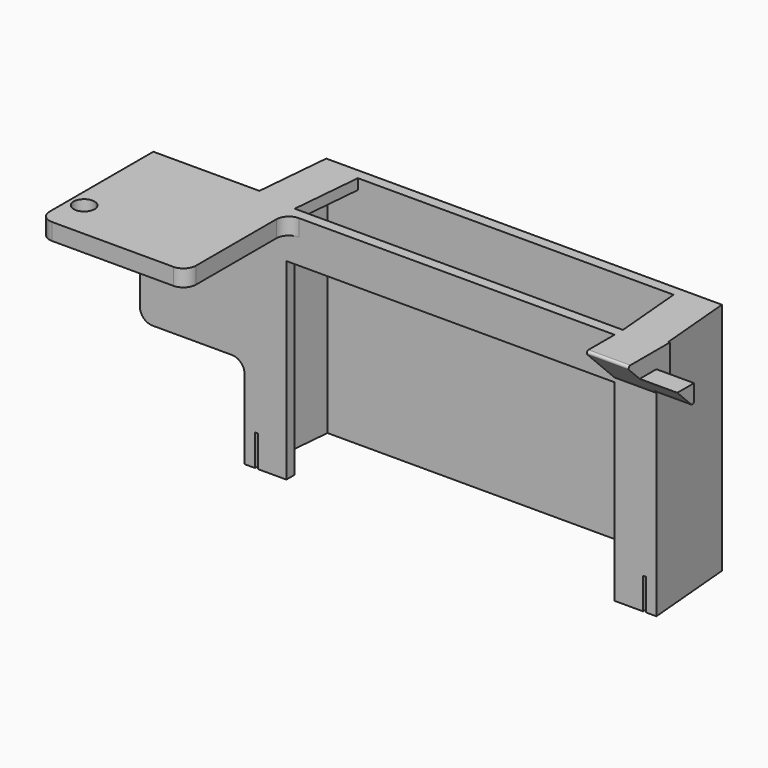
from build123d import *

# Parameters (mm, degrees)
F1_DEPTH     = 56
F3_DEPTH     = 2.5
F5_DEPTH     = 0.75
F6_SIZE      = 0.5
F7_SIZE      = 0.5
F9_DEPTH     = 7.5
F11_DEPTH    = 4
F13_DEPTH    = 30
F15_DEPTH    = 5
F16_W        = 4
F16_H        = 9
F17_DEPTH    = 9
F19_DEPTH    = 10
F20_T1_DEPTH = 25.0355339059
F20_T3_DEPTH = 10.25
F20_T5_DEPTH = 12.017766953
F21_W        = 78.4606024017
F21_H        = 2.5
F22_DEPTH    = 10
F23_R        = 2.5
F24_DEPTH    = 4
F25_R        = 3
F27_DEPTH    = 9


# Not quite as in the source:
# - a fillet or chamfer that OpenCascade refuses, or shapes differently, is made with other operations: its cross-section is extruded or revolved along the edge and cut away or added


with BuildPart() as f1:
    # F0 (on Top) → F1 (new body)
    with BuildSketch(Plane.XY):
        Polygon((-39.2303012009, -8.5), (-46.5, -8.5), (-45, 8.5), (45, 8.5), (46.5, -8.5), (39.2303012009, -8.5), (39.2303012009, -11), (49.2303012009, -11), (47.2891247303, 11), (-47.2891247303, 11), (-49.2303012009, -11), (-39.2303012009, -11), align=None)
    extrude(amount=F1_DEPTH)

    # F2 (on face) → F3 (join)
    with BuildSketch(Plane.XY.offset(56)):
        Polygon((-46.5, -8.5), (-39.2303012009, -8.5), (-37.7303012009, 8.5), (-45, 8.5), align=None)
        Polygon((46.5, -8.5), (45, 8.5), (37.7303012009, 8.5), (39.2303012009, -8.5), align=None)
    extrude(amount=-F3_DEPTH)

    # F4 (on face) → F5 (join)
    with BuildSketch(Plane(origin=(0, 0, 0), x_dir=(1, 0, 0), z_dir=(0, 0, -1))):
        Polygon((-40.7303012009, 7.75), (-40.2303012009, 8.5), (-45.5, 8.5), (-45, 7.75), align=None)
        Polygon((45, 7.75), (45.5, 8.5), (40.2303012009, 8.5), (40.7303012009, 7.75), align=None)
    extrude(amount=-F5_DEPTH)

    # F6
    f6_edges = [f1.edges().sort_by_distance(p)[0] for p in [
        (42.865151, -7.75, 0.75),
    ]]
    chamfer(f6_edges, length=F6_SIZE)

    # F7
    f7_edges = [f1.edges().sort_by_distance(p)[0] for p in [
        (-42.865151, -7.75, 0.75),
    ]]
    chamfer(f7_edges, length=F7_SIZE)

    # F8 (on face) → F9 (cut)
    with BuildSketch(Plane(origin=(0, 0, 0), x_dir=(1, 0, 0), z_dir=(0, 0, -1))):
        Polygon((-46.7205882353, 11), (-46.5, 8.5), (-45.8406183737, 8.5), (-46.061206609, 11), align=None)
        Polygon((46.5, 8.5), (46.7205882353, 11), (46.061206609, 11), (45.8406183737, 8.5), align=None)
    extrude(amount=-F9_DEPTH, mode=Mode.SUBTRACT)

    # F10 (on face) → F11 (join)
    with BuildSketch(Plane.XY.offset(56)):
        Polygon((-74.2303012009, -7), (-74.2303012009, -11), (-74.2303012009, -41), (-39.2303012009, -41), (-39.2303012009, -11), (-49.2303012009, -11), (-48.8773600244, -7), align=None)
        Polygon((49.2303012009, -11), (39.2303012009, -11), (39.2303012009, -20), (58.2303012009, -20), (58.2303012009, -11), (58.2303012009, -7), (48.8773600244, -7), align=None)
    extrude(amount=-F11_DEPTH)

    # F12 (on face) → F13 (join)
    with BuildSketch(Plane(origin=(0, 0, 52), x_dir=(1, 0, 0), z_dir=(0, 0, -1))):
        Polygon((-74.2303012009, 7), (-48.8773600244, 7), (-49.2303012009, 11), (-74.2303012009, 11), align=None)
    extrude(amount=F13_DEPTH)

    # F14 (on face) → F15 (join)
    with BuildSketch(Plane(origin=(0, 0, 52), x_dir=(1, 0, 0), z_dir=(0, 0, -1))):
        Polygon((58.2303012009, 20), (39.2303012009, 20), (39.2303012009, 11), (49.2303012009, 11), (48.8773600244, 7), (58.2303012009, 7), align=None)
    extrude(amount=F15_DEPTH)

    # F16 (on face) → F17 (cut)
    with BuildSketch(Plane.YZ.offset(58.2303012009)):
        Polygon((-11, 47), (-20, 56), (-20, 47), align=None)
        with Locations((-9, 51.5)):
            Rectangle(F16_W, F16_H)
    extrude(amount=-F17_DEPTH, mode=Mode.SUBTRACT)

    # F18 (on face) → F19 (cut)
    with BuildSketch(Plane.YZ.offset(49.2303012009)):
        Polygon((-11, 47), (-20, 56), (-20, 47), align=None)
    extrude(amount=-F19_DEPTH, mode=Mode.SUBTRACT)

    # F20: fillet of radius 0.5 on 3 edges, made by hand

    # F20_s2 → F20_t1 (cut)
    with BuildSketch(Plane.YZ.offset(36.2125342479)):
        with BuildLine():
            ThreePointArc((-19.1464466094, 55.1464466094), (-19.2548329851, 55.6913417162), (-18.7928932188, 56))
            Line((-18.7928932188, 56), (-20, 56))
            Line((-20, 56), (-19.1464466094, 55.1464466094))
        make_face()
    extrude(amount=F20_T1_DEPTH, mode=Mode.SUBTRACT)

    # F20_s4 → F20_t3 (cut)
    with BuildSketch(Plane.YZ.offset(49.2303012009)):
        with BuildLine():
            ThreePointArc((-11, 55.5), (-11.1464466094, 55.8535533906), (-11.5, 56))
            Line((-11.5, 56), (-11, 56))
            Line((-11, 56), (-11, 55.5))
        make_face()
    extrude(amount=F20_T3_DEPTH, mode=Mode.SUBTRACT)

    # F20_s6 → F20_t5 (cut)
    with BuildSketch(Plane.YZ.offset(49.2303012009)):
        with BuildLine():
            ThreePointArc((-11.8535533906, 47.8535533906), (-11.3086582838, 47.7451670149), (-11, 48.2071067812))
            Line((-11, 48.2071067812), (-11, 47))
            Line((-11, 47), (-11.8535533906, 47.8535533906))
        make_face()
    extrude(amount=F20_T5_DEPTH, mode=Mode.SUBTRACT)

    # F21 (on face) → F22 (join)
    with BuildSketch(Plane.XY.offset(56)):
        with Locations((0, -9.75)):
            Rectangle(F21_W, F21_H)
    extrude(amount=-F22_DEPTH)

    # F23 (on face) → F24 (cut)
    with BuildSketch(Plane.XY.offset(56)):
        with Locations((-70.7696987991, -32)):
            Circle(F23_R)
    extrude(amount=-F24_DEPTH, mode=Mode.SUBTRACT)

    # F25
    f25_edges = [f1.edges().sort_by_distance(p)[0] for p in [
        (-74.230301, -41, 54),
        (-39.230301, -41, 54),
        (-74.230301, -9, 22),
        (-49.053831, -9, 22),
        (-39.230301, -11, 54),
    ]]
    fillet(f25_edges, radius=F25_R)

    # F26 (on face) → F27 (cut)
    with BuildSketch(Plane.YZ.offset(58.2303012009)):
        Polygon((-11, 52), (-11, 56), (-20, 56), (-16, 52), align=None)
    extrude(amount=-F27_DEPTH, mode=Mode.SUBTRACT)


solid = f1.part
